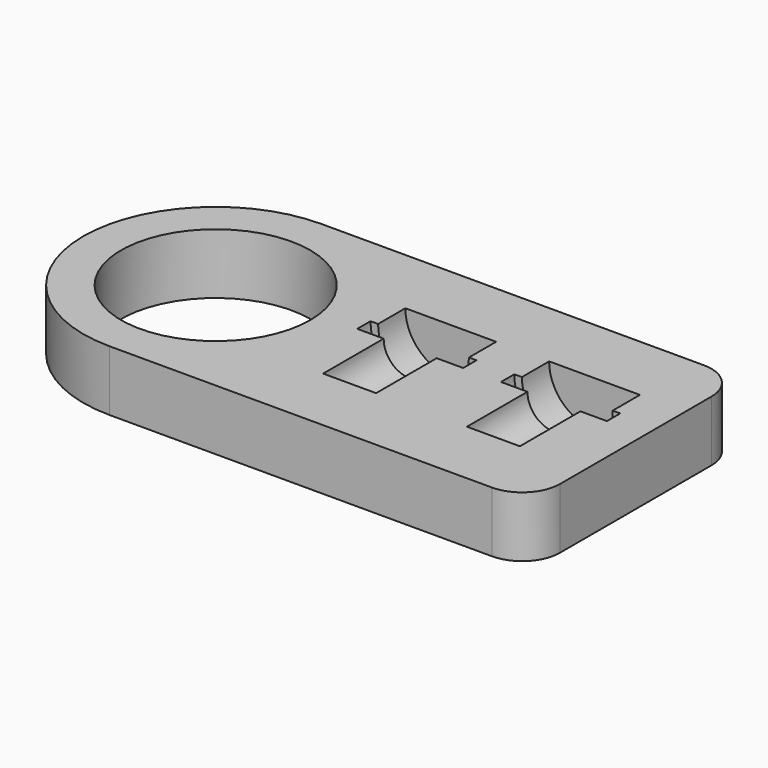
from build123d import *

# Parameters (mm, degrees)
F0_R         = 12.5
F1_DEPTH     = 8
F5_TEXT_SIZE = 5.5555555556
F6_DEPTH     = 1


# Not quite as in the source:
# - Text() gives the source's letters only with a copy of the font that has no kerning and outlines rounded to 1/6400 em; it was checked with that copy


with BuildPart() as f1:
    # F0 (on Top) → F1 (new body)
    with BuildSketch(Plane.XY):
        with BuildLine():
            ThreePointArc((0, 17.5), (5.1256313292, 5.1256313292), (17.5, 0))
            Line((17.5, 0), (68, 0))
            ThreePointArc((68, 0), (71.5355339059, 1.4644660941), (73, 5))
            Line((73, 5), (73, 30))
            ThreePointArc((73, 30), (71.5355339059, 33.5355339059), (68, 35))
            Line((68, 35), (17.5, 35))
            ThreePointArc((17.5, 35), (5.1256313292, 29.8743686708), (0, 17.5))
        make_face()
        with Locations((17.5, 17.5)):
            Circle(F0_R, mode=Mode.SUBTRACT)
    extrude(amount=F1_DEPTH)

    # F2 (on face) → F3 (revolve, cut)
    with BuildSketch(Plane.XY.offset(8)):
        Polygon((42, 19), (42, 9), (45.5, 9), (45.5, 19), (49, 19), (49, 21.2), (48, 21.2), (48, 25.7), (42, 25.7), (42, 21.2), align=None)
    revolve(axis=Axis((42, 14, 8), (0, 1, 0)), mode=Mode.SUBTRACT)

    # F2 (on face) → F4 (revolve, cut)
    with BuildSketch(Plane.XY.offset(8)):
        Polygon((61, 19), (61, 9), (64.5, 9), (64.5, 19), (68, 19), (68, 21.2), (67, 21.2), (67, 25.7), (61, 25.7), (61, 21.2), align=None)
    revolve(axis=Axis((61, 14, 8), (0, 1, 0)), mode=Mode.SUBTRACT)

    # F5 (on face) → F6 (cut)
    with BuildSketch(Plane(origin=(0, 0, 0), x_dir=(1, 0, 0), z_dir=(0, 0, -1))):
        with Locations((30, -9)):
            Text('814, 815', F5_TEXT_SIZE, font='Open Sans', text_align=(TextAlign.LEFT, TextAlign.BOTTOM))
    extrude(amount=-F6_DEPTH, mode=Mode.SUBTRACT)


solid = f1.part
